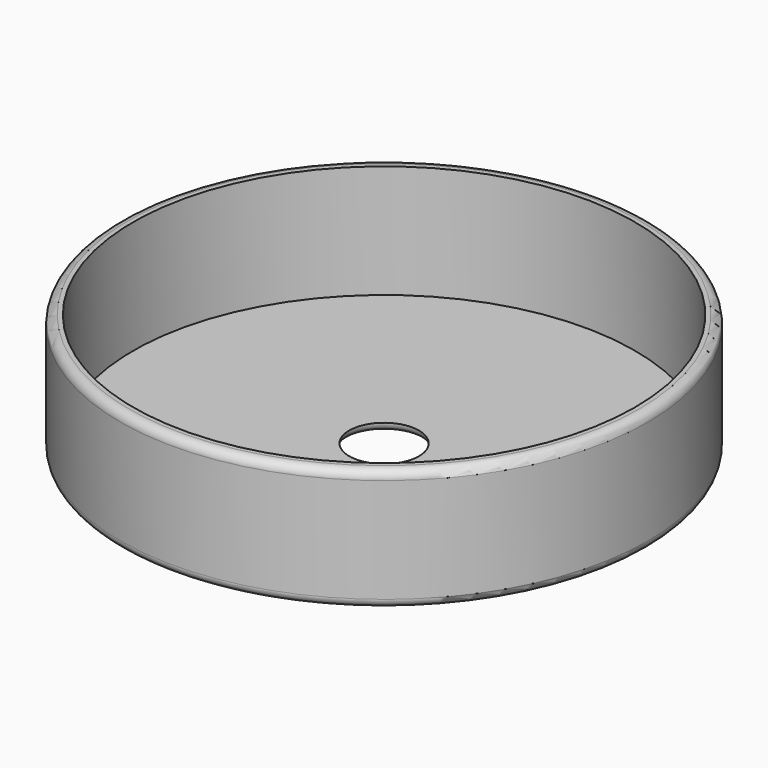
from build123d import *

# Parameters (mm, degrees)
F0_R     = 30.3
F1_DEPTH = 14
F2_R     = 28.8
F3_DEPTH = 13
F4_R     = 4
F5_DEPTH = 25.4
F6_R     = 0.99999


# Not quite as in the source:
# - a fillet or chamfer is up to 0.001 mm smaller than in the source, because OpenCascade refuses the exact size


with BuildPart() as f1:
    # F0 (on Top) → F1 (new body)
    with BuildSketch(Plane.XY):
        Circle(F0_R)
    extrude(amount=F1_DEPTH)

    # F2 (on face) → F3 (cut)
    with BuildSketch(Plane.XY.offset(14)):
        Circle(F2_R)
    extrude(amount=-F3_DEPTH, mode=Mode.SUBTRACT)

    # F4 (on face) → F5 (cut)
    with BuildSketch(Plane.XY.offset(1)):
        Circle(F4_R)
    extrude(amount=-F5_DEPTH, mode=Mode.SUBTRACT)

    # F6 (radius 1 in the source; OpenCascade refuses exactly that, so slightly less here)
    f6_edges = [f1.edges().sort_by_distance(p)[0] for p in [
        (-30.3, 0, 0),
        (-4, 0, 0),
        (-30.3, 0, 14),
    ]]
    fillet(f6_edges, radius=F6_R)


solid = f1.part
